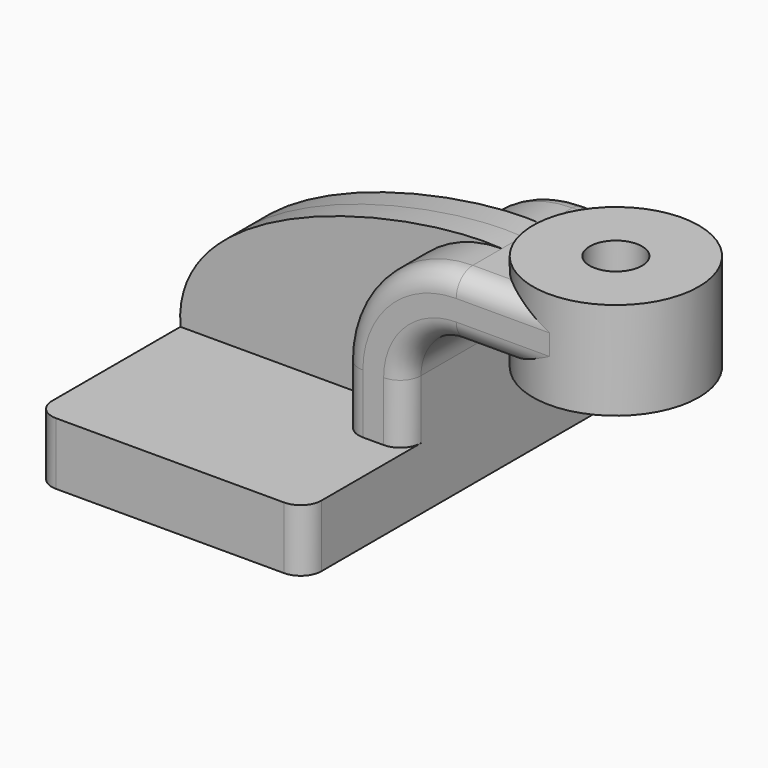
from build123d import *

# Parameters (mm, degrees)
F1_DEPTH     = 63.5
F0_W         = 25.4
F0_H         = 19.05
F2_DEPTH     = 25.4
F3_DEPTH     = 7.9375
F5_T1_DEPTH  = 50.8
F5_T3_DEPTH  = 18.1687793255
F5_T6_ANGLE  = 90
F5_T8_ANGLE  = 90
F5_T10_ANGLE = 90
F5_T12_ANGLE = 90
F5_T16_DEPTH = 55.5625
F5_S17_R     = 25.4
F5_T18_DEPTH = 30
F5_T22_DEPTH = 55.5625
F5_S23_R     = 25.4
F5_T24_DEPTH = 30
F5_T28_DEPTH = 55.5625
F5_S29_R     = 25.4
F5_T30_DEPTH = 30
F5_T34_DEPTH = 55.5625
F5_S35_R     = 25.4
F5_T36_DEPTH = 30
F6_R         = 8.0264807454
F7_DEPTH     = 12.7
F8_D         = 10
F8_DEPTH     = 63.501


# Not quite as in the source:
# - a fillet or chamfer that OpenCascade refuses, or shapes differently, is made with other operations: its cross-section is extruded or revolved along the edge and cut away or added


with BuildPart() as f1:
    # F0 (on Front) → F1 (new body, symmetric)
    with BuildSketch(Plane.XZ):
        Polygon((-82.55, 0), (0, 0), (0, 19.05), (-19.05, 19.05), (-82.55, 19.05), align=None)
    extrude(amount=F1_DEPTH, both=True)

    # F0 (on Front) → F2 (join, symmetric)
    with BuildSketch(Plane.XZ):
        with BuildLine():
            Line((-19.05, 19.05), (0, 19.05))
            Line((0, 19.05), (0, 37.2187793255))
            ThreePointArc((0, 37.2187793255), (4.6496798487, 48.4440994768), (15.875, 53.0937793255))
            Line((15.875, 53.0937793255), (19.05, 53.0937793255))
            Line((19.05, 53.0937793255), (19.05, 72.1437793255))
            Line((19.05, 72.1437793255), (15.875, 72.1437793255))
            ThreePointArc((15.875, 72.1437793255), (-8.8207043329, 61.9144836584), (-19.05, 37.2187793255))
            Line((-19.05, 37.2187793255), (-19.05, 19.05))
        make_face()
        with Locations((31.75, 62.6187793255)):
            Rectangle(F0_W, F0_H)
    extrude(amount=F2_DEPTH, both=True)

    # F0 (on Front) → F3 (join, symmetric)
    with BuildSketch(Plane.XZ):
        with BuildLine():
            add(Edge.make_bspline(
                [(-82.55, 19.05), (-85.6057107449, 57.0069514215), (-12.4422926456, 74.3687301874), (15.875, 72.1437793255)],
                knots=[0, 0, 0, 0, 111.8321511376, 111.8321511376, 111.8321511376, 111.8321511376], degree=3))
            Line((-82.55, 19.05), (-19.05, 19.05))
            Line((-19.05, 19.05), (-19.05, 37.2187793255))
            ThreePointArc((-19.05, 37.2187793255), (-8.8207043329, 61.9144836584), (15.875, 72.1437793255))
        make_face()
    extrude(amount=F3_DEPTH, both=True)

    # F0 (on Front) → F4 (revolve)
    with BuildSketch(Plane.XZ):
        Polygon((44.45, 76.2), (44.45, 72.1437793255), (44.45, 53.0937793255), (44.45, 46.355), (69.85, 46.355), (69.85, 76.2), align=None)
    revolve(axis=Axis((44.45, 0, 61.2775), (0, 0, 1)))

    # F5: fillet of radius 6.35 on 12 edges, made by hand

    # F5_s2 → F5_t1 (cut)
    with BuildSketch(Plane.XY.offset(-15.875)):
        with BuildLine():
            ThreePointArc((-76.2, -63.5), (-80.6901280605, -61.6401280605), (-82.55, -57.15))
            Line((-82.55, -57.15), (-82.55, -63.5))
            Line((-82.55, -63.5), (-76.2, -63.5))
        make_face()
        with BuildLine():
            ThreePointArc((0, -57.15), (-1.8598719395, -61.6401280605), (-6.35, -63.5))
            Line((-6.35, -63.5), (0, -63.5))
            Line((0, -63.5), (0, -57.15))
        make_face()
        with BuildLine():
            ThreePointArc((-76.2, 63.5), (-80.6901280605, 61.6401280605), (-82.55, 57.15))
            Line((-82.55, 57.15), (-82.55, 63.5))
            Line((-82.55, 63.5), (-76.2, 63.5))
        make_face()
        with BuildLine():
            ThreePointArc((-6.35, 63.5), (-1.8598719395, 61.6401280605), (0, 57.15))
            Line((0, 57.15), (0, 63.5))
            Line((0, 63.5), (-6.35, 63.5))
        make_face()
    extrude(amount=F5_T1_DEPTH, mode=Mode.SUBTRACT)

    # F5_s4 → F5_t3 (cut)
    with BuildSketch(Plane.XY.offset(19.05)):
        with BuildLine():
            ThreePointArc((-12.7, 25.4), (-17.1901280605, 23.5401280605), (-19.05, 19.05))
            Line((-19.05, 19.05), (-19.05, 25.4))
            Line((-19.05, 25.4), (-12.7, 25.4))
        make_face()
        with BuildLine():
            ThreePointArc((-12.7, -25.4), (-17.1901280605, -23.5401280605), (-19.05, -19.05))
            Line((-19.05, -19.05), (-19.05, -25.4))
            Line((-19.05, -25.4), (-12.7, -25.4))
        make_face()
        with BuildLine():
            ThreePointArc((0, 19.05), (-1.8598719395, 23.5401280605), (-6.35, 25.4))
            Line((-6.35, 25.4), (0, 25.4))
            Line((0, 25.4), (0, 19.05))
        make_face()
        with BuildLine():
            ThreePointArc((0, -19.05), (-1.8598719395, -23.5401280605), (-6.35, -25.4))
            Line((-6.35, -25.4), (0, -25.4))
            Line((0, -25.4), (0, -19.05))
        make_face()
    extrude(amount=F5_T3_DEPTH, mode=Mode.SUBTRACT)

    # F5_s5 → F5_t6 (revolve, cut)
    with BuildSketch(Plane.XY.offset(37.2187793255)):
        with BuildLine():
            ThreePointArc((-6.35, 25.4), (-1.8598719395, 23.5401280605), (0, 19.05))
            Line((0, 19.05), (0, 25.4))
            Line((0, 25.4), (-6.35, 25.4))
        make_face()
    revolve(axis=Axis((15.875, 25.4, 37.2187793255), (0, 1, 0)), revolution_arc=F5_T6_ANGLE, mode=Mode.SUBTRACT)

    # F5_s7 → F5_t8 (revolve, cut)
    with BuildSketch(Plane.YZ.offset(15.875)):
        with BuildLine():
            ThreePointArc((25.4, 65.7937793255), (23.5401280605, 70.283907386), (19.05, 72.1437793255))
            Line((19.05, 72.1437793255), (25.4, 72.1437793255))
            Line((25.4, 72.1437793255), (25.4, 65.7937793255))
        make_face()
    revolve(axis=Axis((15.875, 25.4, 37.2187793255), (0, -1, 0)), revolution_arc=F5_T8_ANGLE, mode=Mode.SUBTRACT)

    # F5_s9 → F5_t10 (revolve, cut)
    with BuildSketch(Plane.XY.offset(37.2187793255)):
        with BuildLine():
            ThreePointArc((0, -19.05), (-1.8598719395, -23.5401280605), (-6.35, -25.4))
            Line((-6.35, -25.4), (0, -25.4))
            Line((0, -25.4), (0, -19.05))
        make_face()
    revolve(axis=Axis((15.875, -25.4, 37.2187793255), (0, 1, 0)), revolution_arc=F5_T10_ANGLE, mode=Mode.SUBTRACT)

    # F5_s11 → F5_t12 (revolve, cut)
    with BuildSketch(Plane.YZ.offset(15.875)):
        with BuildLine():
            ThreePointArc((-25.4, 65.7937793255), (-23.5401280605, 70.283907386), (-19.05, 72.1437793255))
            Line((-19.05, 72.1437793255), (-25.4, 72.1437793255))
            Line((-25.4, 72.1437793255), (-25.4, 65.7937793255))
        make_face()
    revolve(axis=Axis((15.875, -25.4, 37.2187793255), (0, -1, 0)), revolution_arc=F5_T12_ANGLE, mode=Mode.SUBTRACT)


with BuildPart() as f5_tool14:
    # F5_s15 → F5_t16 (new body)
    with BuildSketch(Plane.YZ.offset(71.4375)):
        with BuildLine():
            ThreePointArc((-25.4, 65.7937793255), (-23.5401280605, 70.283907386), (-19.05, 72.1437793255))
            Line((-19.05, 72.1437793255), (-25.4, 72.1437793255))
            Line((-25.4, 72.1437793255), (-25.4, 65.7937793255))
        make_face()
    extrude(amount=-F5_T16_DEPTH)

    # F5_s17 → F5_t18 (cut, symmetric)
    with BuildSketch(Plane.XY.offset(69)):
        with Locations((44.45, 0)):
            Circle(F5_S17_R)
    extrude(amount=F5_T18_DEPTH, both=True, mode=Mode.SUBTRACT)


with BuildPart() as f1_1:
    add(f1.part)

    # F5_t13: cut F5_tool14
    add(f5_tool14.part, mode=Mode.SUBTRACT)


with BuildPart() as f5_tool20:
    # F5_s21 → F5_t22 (new body)
    with BuildSketch(Plane.YZ.offset(15.875)):
        with BuildLine():
            ThreePointArc((-25.4, 59.4437793255), (-23.5401280605, 54.953651265), (-19.05, 53.0937793255))
            Line((-19.05, 53.0937793255), (-25.4, 53.0937793255))
            Line((-25.4, 53.0937793255), (-25.4, 59.4437793255))
        make_face()
    extrude(amount=F5_T22_DEPTH)

    # F5_s23 → F5_t24 (cut, symmetric)
    with BuildSketch(Plane.XY.offset(56.3)):
        with Locations((44.45, 0)):
            Circle(F5_S23_R)
    extrude(amount=F5_T24_DEPTH, both=True, mode=Mode.SUBTRACT)


with BuildPart() as f1_2:
    add(f1_1.part)

    # F5_t19: cut F5_tool20
    add(f5_tool20.part, mode=Mode.SUBTRACT)


with BuildPart() as f5_tool26:
    # F5_s27 → F5_t28 (new body)
    with BuildSketch(Plane.YZ.offset(71.4375)):
        with BuildLine():
            ThreePointArc((25.4, 65.7937793255), (23.5401280605, 70.283907386), (19.05, 72.1437793255))
            Line((19.05, 72.1437793255), (25.4, 72.1437793255))
            Line((25.4, 72.1437793255), (25.4, 65.7937793255))
        make_face()
    extrude(amount=-F5_T28_DEPTH)

    # F5_s29 → F5_t30 (cut, symmetric)
    with BuildSketch(Plane.XY.offset(69)):
        with Locations((44.45, 0)):
            Circle(F5_S29_R)
    extrude(amount=F5_T30_DEPTH, both=True, mode=Mode.SUBTRACT)


with BuildPart() as f1_3:
    add(f1_2.part)

    # F5_t25: cut F5_tool26
    add(f5_tool26.part, mode=Mode.SUBTRACT)


with BuildPart() as f5_tool32:
    # F5_s33 → F5_t34 (new body)
    with BuildSketch(Plane.YZ.offset(15.875)):
        with BuildLine():
            ThreePointArc((25.4, 59.4437793255), (23.5401280605, 54.953651265), (19.05, 53.0937793255))
            Line((19.05, 53.0937793255), (25.4, 53.0937793255))
            Line((25.4, 53.0937793255), (25.4, 59.4437793255))
        make_face()
    extrude(amount=F5_T34_DEPTH)

    # F5_s35 → F5_t36 (cut, symmetric)
    with BuildSketch(Plane.XY.offset(56.3)):
        with Locations((44.45, 0)):
            Circle(F5_S35_R)
    extrude(amount=F5_T36_DEPTH, both=True, mode=Mode.SUBTRACT)


with BuildPart() as f1_4:
    add(f1_3.part)

    # F5_t31: cut F5_tool32
    add(f5_tool32.part, mode=Mode.SUBTRACT)

    # F6 (on face) → F7 (cut)
    with BuildSketch(Plane.XY.offset(76.2)):
        with Locations((44.45, 0)):
            Circle(F6_R)
    extrude(amount=-F7_DEPTH, mode=Mode.SUBTRACT)

    # F8 (through all, one way)
    with BuildSketch(Plane.XZ):
        with Locations((44.45, 61.2775)):
            Circle(F8_D / 2)
    extrude(amount=-F8_DEPTH, mode=Mode.SUBTRACT)


solid = f1_4.part
